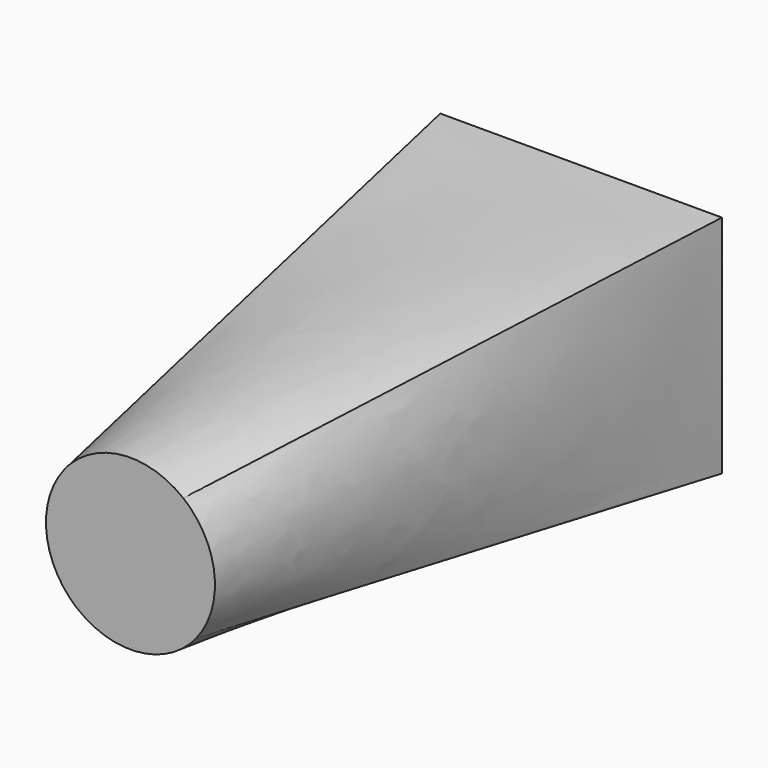
from build123d import *

# Parameters (mm, degrees)
F0_W = 100
F0_H = 80
F4_T = 2


# Not quite as in the source:
# - the arcs of a loft's sections are written as splines that run evenly, so that the points pair up as in the source's solid
# - a shell that OpenCascade refuses in one call is made with other operations: the cavity is built on its own and cut out


with BuildPart() as f3:
    # F0 (on Front) → F3 section 0
    with BuildSketch(Plane.XZ):
        Rectangle(F0_W, F0_H)
    # F2 (on offset) → F3 section 1
    with BuildSketch(Plane.XZ.offset(200)):
        with BuildLine():
            add(Edge.make_bspline(
                [(23.4260642833, -18.7408514266), (24.6526501409, -17.2076191047), (25.7281991997, -15.5536195196), (27.5359963334, -12.0674860741), (28.2681997069, -10.2354384151), (29.3611496291, -6.4636063212), (29.7218691524, -4.5239151524), (30.0579704105, -0.6113338023), (30.0333438346, 1.3614596326), (29.5996802458, 5.2644319319), (29.1906539561, 7.1945142875), (28.0038909689, 10.9378884992), (27.2261836164, 12.751087793), (25.3319278668, 16.1910081455), (24.215426309, 17.8176441455), (21.6864729832, 20.8219164288), (20.2740837486, 22.1994784257), (18.7408514266, 23.4260642833)],
                knots=[0, 0, 0, 0, 0.125, 0.125, 0.25, 0.25, 0.375, 0.375, 0.5, 0.5, 0.625, 0.625, 0.75, 0.75, 0.875, 0.875, 1, 1, 1, 1], degree=3))
            add(Edge.make_bspline(
                [(18.7408514266, 23.4260642833), (17.2076191047, 24.6526501409), (15.5536195196, 25.7281991997), (12.0674860741, 27.5359963334), (10.2354384151, 28.2681997069), (6.4636063212, 29.3611496291), (4.5239151524, 29.7218691524), (0.6113338023, 30.0579704105), (-1.3614596326, 30.0333438346), (-5.2644319319, 29.5996802458), (-7.1945142875, 29.1906539561), (-10.9378884992, 28.0038909689), (-12.751087793, 27.2261836164), (-16.1910081455, 25.3319278668), (-17.8176441455, 24.215426309), (-20.8219164288, 21.6864729832), (-22.1994784257, 20.2740837486), (-23.4260642833, 18.7408514266)],
                knots=[0, 0, 0, 0, 0.125, 0.125, 0.25, 0.25, 0.375, 0.375, 0.5, 0.5, 0.625, 0.625, 0.75, 0.75, 0.875, 0.875, 1, 1, 1, 1], degree=3))
            add(Edge.make_bspline(
                [(-23.4260642833, 18.7408514266), (-24.6526501409, 17.2076191047), (-25.7281991997, 15.5536195196), (-27.5359963334, 12.0674860741), (-28.2681997069, 10.2354384151), (-29.3611496291, 6.4636063212), (-29.7218691524, 4.5239151524), (-30.0579704105, 0.6113338023), (-30.0333438346, -1.3614596326), (-29.5996802458, -5.2644319319), (-29.1906539561, -7.1945142875), (-28.0038909689, -10.9378884992), (-27.2261836164, -12.751087793), (-25.3319278668, -16.1910081455), (-24.215426309, -17.8176441455), (-21.6864729832, -20.8219164288), (-20.2740837486, -22.1994784257), (-18.7408514266, -23.4260642833)],
                knots=[0, 0, 0, 0, 0.125, 0.125, 0.25, 0.25, 0.375, 0.375, 0.5, 0.5, 0.625, 0.625, 0.75, 0.75, 0.875, 0.875, 1, 1, 1, 1], degree=3))
            add(Edge.make_bspline(
                [(-18.7408514266, -23.4260642833), (-17.2076191047, -24.6526501409), (-15.5536195196, -25.7281991997), (-12.0674860741, -27.5359963334), (-10.2354384151, -28.2681997069), (-6.4636063212, -29.3611496291), (-4.5239151524, -29.7218691524), (-0.6113338023, -30.0579704105), (1.3614596326, -30.0333438346), (5.2644319319, -29.5996802458), (7.1945142875, -29.1906539561), (10.9378884992, -28.0038909689), (12.751087793, -27.2261836164), (16.1910081455, -25.3319278668), (17.8176441455, -24.215426309), (20.8219164288, -21.6864729832), (22.1994784257, -20.2740837486), (23.4260642833, -18.7408514266)],
                knots=[0, 0, 0, 0, 0.125, 0.125, 0.25, 0.25, 0.375, 0.375, 0.5, 0.5, 0.625, 0.625, 0.75, 0.75, 0.875, 0.875, 1, 1, 1, 1], degree=3))
        make_face()
    loft(ruled=True)

    # F4: shell of thickness 2, made by hand


with BuildPart() as f4_core1:
    # F4_t2: copy of F3
    add(f3.part)

    # the walls: a layer under each face that stays
    f4_faces = [f4_core1.faces().sort_by_distance(p)[0] for p in [
        (1.6564728911, -100, -34.9082560201),
        (39.9082560201, -100, 1.6564728911),
        (-1.6564728911, -100, 34.9082560201),
        (-39.9082560201, -100, -1.6564728911),
        (0, -200, 0),
    ]]
    thicken(f4_faces, amount=-F4_T, mode=Mode.SUBTRACT)


with BuildPart() as f3_1:
    add(f3.part)

    # what is left inside the walls is the cavity
    f4_cavity = [f4_core1.part.solids().sort_by_distance(p)[0] for p in [
        (-1.053831, -66.075437, 34.613436),
    ]]
    add(f4_cavity, mode=Mode.SUBTRACT)


solid = f3_1.part
